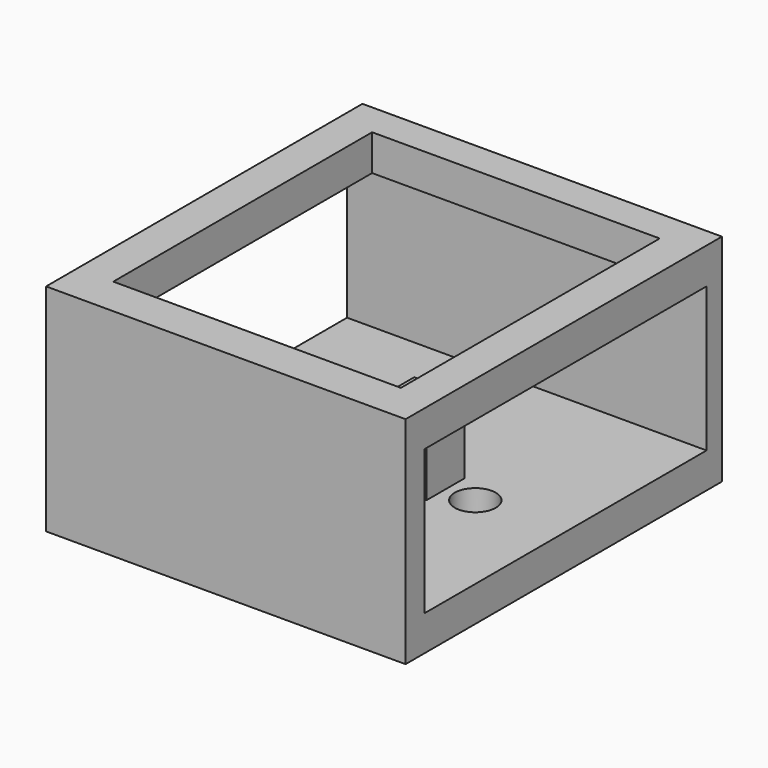
from build123d import *

# Parameters (mm, degrees)
F2_W     = 50
F2_H     = 55
F3_DEPTH = 30
F4_W     = 49
F4_H     = 20.1
F5_DEPTH = 50.001
F0_R     = 2.85
F6_DEPTH = 4.9
F0_W     = 7
F0_H     = 6.6
F7_DEPTH = 15
F8_START = 25
F1_W     = 40
F1_H     = 45
F8_DEPTH = 25


# Not quite as in the source:
# - a feature names something its author has since deleted; it is built from what else it names


with BuildPart() as f3:
    # F2 (on Top) → F3 (new body)
    with BuildSketch(Plane.XY):
        with Locations((-48.7460665315, -28.1598071134)):
            Rectangle(F2_W, F2_H)
    extrude(amount=F3_DEPTH)

    # F4 (on face) → F5 (cut, through all)
    with BuildSketch(Plane.YZ.offset(-23.7460665315)):
        with Locations((-27.83, 14.95)):
            Rectangle(F4_W, F4_H)
    extrude(amount=-F5_DEPTH, mode=Mode.SUBTRACT)

    # F0 (on Top) → F6 (cut, through all)
    with BuildSketch(Plane.XY):
        with Locations((-36.0460665315, -28.1598071134)):
            Circle(F0_R)
        with Locations((-61.4460665315, -28.1598071134)):
            Circle(F0_R)
    extrude(amount=F6_DEPTH, mode=Mode.SUBTRACT)

    # F0 (on Top) → F7 (join)
    with BuildSketch(Plane.XY):
        with Locations((-43.6801504195, -28.1598071134)):
            Rectangle(F0_W, F0_H)
    extrude(amount=F7_DEPTH)

    # F1 (on Top) → F8 (cut)
    with BuildSketch(Plane.XY.offset(F8_START)):
        with Locations((-48.7460665315, -27.7248071134)):
            Rectangle(F1_W, F1_H)
    extrude(amount=F8_DEPTH, mode=Mode.SUBTRACT)


solid = f3.part
